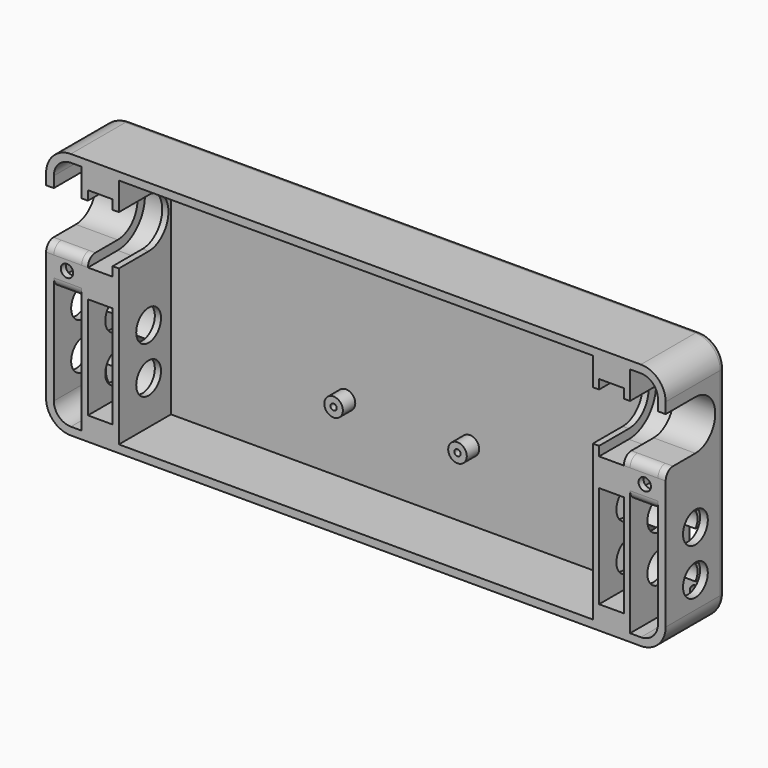
from build123d import *

# Parameters (mm, degrees)
F1_DEPTH  = 24
F3_DEPTH  = 21
F4_R      = 2
F5_R      = 2
F5_W      = 9
F5_H      = 57
F5_W_2    = 8
F5_H_2    = 75
F6_DEPTH  = 3.001
F7_W      = 2
F7_H      = 75
F8_DEPTH  = 21
F9_R      = 5
F10_DEPTH = 200.001
F12_DEPTH = 9
F13_W     = 56.962027
F13_H     = 98.82912
F14_DEPTH = 100.001
F15_R     = 3
F16_R     = 2
F17_DEPTH = 24.001
F18_R     = 3
F18_R_2   = 1
F19_DEPTH = 5
F21_DEPTH = 8


with BuildPart() as f1:
    # F0 (on Front) → F1 (new body)
    with BuildSketch(Plane.XZ):
        with BuildLine():
            Line((-92, -40), (92, -40))
            ThreePointArc((92, -40), (97.656854, -37.656854), (100, -32))
            Line((100, -32), (100, 32))
            ThreePointArc((100, 32), (97.656854, 37.656854), (92, 40))
            Line((92, 40), (-92, 40))
            ThreePointArc((-92, 40), (-97.656854, 37.656854), (-100, 32))
            Line((-100, 32), (-100, -32))
            ThreePointArc((-100, -32), (-97.656854, -37.656854), (-92, -40))
        make_face()
    extrude(amount=F1_DEPTH)

    # F2 (on face) → F3 (cut)
    with BuildSketch(Plane.XZ.offset(24)):
        with BuildLine():
            ThreePointArc((92, -37.5), (95.889087, -35.889087), (97.5, -32))
            Line((97.5, -32), (97.5, 32))
            ThreePointArc((97.5, 32), (95.889087, 35.889087), (92, 37.5))
            Line((92, 37.5), (-92, 37.5))
            ThreePointArc((-92, 37.5), (-95.889087, 35.889087), (-97.5, 32))
            Line((-97.5, 32), (-97.5, -32))
            ThreePointArc((-97.5, -32), (-95.889087, -35.889087), (-92, -37.5))
            Line((-92, -37.5), (92, -37.5))
        make_face()
    extrude(amount=-F3_DEPTH, mode=Mode.SUBTRACT)

    # F4
    f4_edges = [f1.edges().sort_by_distance(p)[0] for p in [
        (0, 0, 40),
    ]]
    fillet(f4_edges, radius=F4_R)

    # F5 (on face) → F6 (cut, through all)
    with BuildSketch(Plane.XZ.offset(3)):
        with Locations((-93, 33)):
            Circle(F5_R)
        with Locations((93, 33)):
            Circle(F5_R)
        with Locations((-93, -33)):
            Circle(F5_R)
        with Locations((93, -33)):
            Circle(F5_R)
        with Locations((-93, 0)):
            Rectangle(F5_W, F5_H)
        with Locations((93, 0)):
            Rectangle(F5_W, F5_H)
        with Locations((-82.5, 0)):
            Rectangle(F5_W_2, F5_H_2)
    extrude(amount=-F6_DEPTH, mode=Mode.SUBTRACT)

    # F7 (on face) → F8 (join, through all)
    with BuildSketch(Plane.XZ.offset(3)):
        with Locations((-87.5, 0)):
            Rectangle(F7_W, F7_H)
        with Locations((87.5, 0)):
            Rectangle(F7_W, F7_H)
        with Locations((-77.5, 0)):
            Rectangle(F7_W, F7_H)
        with Locations((77.5, 0)):
            Rectangle(F7_W, F7_H)
    extrude(amount=F8_DEPTH)

    # F9 (on face) → F10 (cut, through all)
    with BuildSketch(Plane(origin=(-100, 0, 0), x_dir=(0, -1, 0), z_dir=(-1, 0, 0))):
        with BuildLine():
            Line((24, 28.5), (12, 28.5))
            ThreePointArc((12, 28.5), (4, 20.5), (12, 12.5))
            Line((12, 12.5), (24, 12.5))
            Line((24, 12.5), (24, 28.5))
        make_face()
        with Locations((12, -23.5)):
            Circle(F9_R)
        with Locations((12, -8.5)):
            Circle(F9_R)
    extrude(amount=-F10_DEPTH, mode=Mode.SUBTRACT)

    # F11 (on face) → F12 (join, through all)
    with BuildSketch(Plane(origin=(-88.5, 0, 0), x_dir=(0, -1, 0), z_dir=(-1, 0, 0))):
        with BuildLine():
            ThreePointArc((8.877501, -26), (8, -23.5), (8.877501, -21))
            Line((8.877501, -21), (6, -21))
            ThreePointArc((6, -21), (4.585786, -21.585786), (4, -23))
            Line((4, -23), (4, -24))
            ThreePointArc((4, -24), (4.585786, -25.414214), (6, -26))
            Line((6, -26), (8.877501, -26))
        make_face()
        with BuildLine():
            ThreePointArc((4, -9), (4.585786, -10.414214), (6, -11))
            Line((6, -11), (8.877501, -11))
            ThreePointArc((8.877501, -11), (8, -8.5), (8.877501, -6))
            Line((8.877501, -6), (6, -6))
            ThreePointArc((6, -6), (4.585786, -6.585786), (4, -8))
            Line((4, -8), (4, -9))
        make_face()
        with BuildLine():
            Line((0, 2), (0, 0))
            Line((0, 0), (21, 0))
            ThreePointArc((21, 0), (23.12132, 0.87868), (24, 3))
            Line((24, 3), (24, 9.5))
            ThreePointArc((24, 9.5), (23.12132, 11.62132), (21, 12.5))
            Line((21, 12.5), (12, 12.5))
            ThreePointArc((12, 12.5), (4, 20.5), (12, 28.5))
            Line((12, 28.5), (3, 28.5))
            Line((3, 28.5), (0, 28.5))
            Line((0, 28.5), (0, 26.5))
            Line((0, 26.5), (3, 26.5))
            Line((3, 26.5), (3.999999, 26.5))
            ThreePointArc((3.999999, 26.5), (3.055728, 16.027864), (12, 10.5))
            Line((12, 10.5), (21, 10.5))
            ThreePointArc((21, 10.5), (21.707107, 10.207107), (22, 9.5))
            Line((22, 9.5), (22, 3))
            ThreePointArc((22, 3), (21.707107, 2.292893), (21, 2))
            Line((21, 2), (0, 2))
        make_face()
    extrude(amount=F12_DEPTH)

    # F13 (on Right) → F14 (cut, through all)
    with BuildSketch(Plane.YZ):
        with Locations((-13.528482, -2.136078)):
            Rectangle(F13_W, F13_H)
    extrude(amount=F14_DEPTH, mode=Mode.SUBTRACT)

    # F15
    f15_edges = [f1.edges().sort_by_distance(p)[0] for p in [
        (-98.75, -24, 12.5),
        (-87.5, -24, 12.5),
    ]]
    fillet(f15_edges, radius=F15_R)

    # F16 (on face) → F17 (cut, through all)
    with BuildSketch(Plane.XZ.offset(24)):
        with Locations((-93.25, 6.36502)):
            Circle(F16_R)
    extrude(amount=-F17_DEPTH, mode=Mode.SUBTRACT)

    # F18 (on face) → F19 (join)
    with BuildSketch(Plane.XZ.offset(3)):
        with Locations((-20, -15)):
            Circle(F18_R)
        with Locations((-20, -15)):
            Circle(F18_R_2, mode=Mode.SUBTRACT)
    extrude(amount=F19_DEPTH)

    # F20 (on face) → F21 (join, through all)
    with BuildSketch(Plane(origin=(-78.5, 0, 0), x_dir=(0, -1, 0), z_dir=(-1, 0, 0))):
        with BuildLine():
            ThreePointArc((12, 33.5), (-1, 20.5), (12, 7.5))
            Line((12, 7.5), (22, 7.5))
            Line((22, 7.5), (22, 2.5))
            Line((22, 2.5), (12, 2.5))
            ThreePointArc((12, 2.5), (7.334678, 1.461665), (3.550114, -1.457314))
            Line((3.550114, -1.457314), (0, -5.716777))
            Line((0, -5.716777), (0, -26.283223))
            Line((0, -26.283223), (3.550114, -30.542686))
            ThreePointArc((3.550114, -30.542686), (7.334678, -33.461665), (12, -34.5))
            Line((12, -34.5), (22, -34.5))
            Line((22, -34.5), (22, -37.5))
            Line((22, -37.5), (24, -37.5))
            Line((24, -37.5), (24, -34.5))
            Line((24, -34.5), (24, -32.5))
            Line((24, -32.5), (12, -32.5))
            ThreePointArc((12, -32.5), (3.383156, -26.098076), (7.025063, -16))
            ThreePointArc((7.025063, -16), (3.383156, -5.901924), (12, 0.5))
            Line((12, 0.5), (24, 0.5))
            Line((24, 0.5), (24, 2.5))
            Line((24, 2.5), (24, 7.5))
            Line((24, 7.5), (24, 9.5))
            Line((24, 9.5), (12, 9.5))
            ThreePointArc((12, 9.5), (1, 20.5), (12, 31.5))
            Line((12, 31.5), (24, 31.5))
            Line((24, 31.5), (24, 32.5))
            Line((24, 32.5), (24, 33.5))
            Line((24, 33.5), (24, 37.5))
            Line((24, 37.5), (22, 37.5))
            Line((22, 37.5), (22, 33.5))
            Line((22, 33.5), (12, 33.5))
        make_face()
    extrude(amount=F21_DEPTH)

    # F22: F1 across plane


with BuildPart() as f1_1:
    add(f1.part)
    add(f1.part.mirror(Plane.YZ))


solid = f1_1.part
